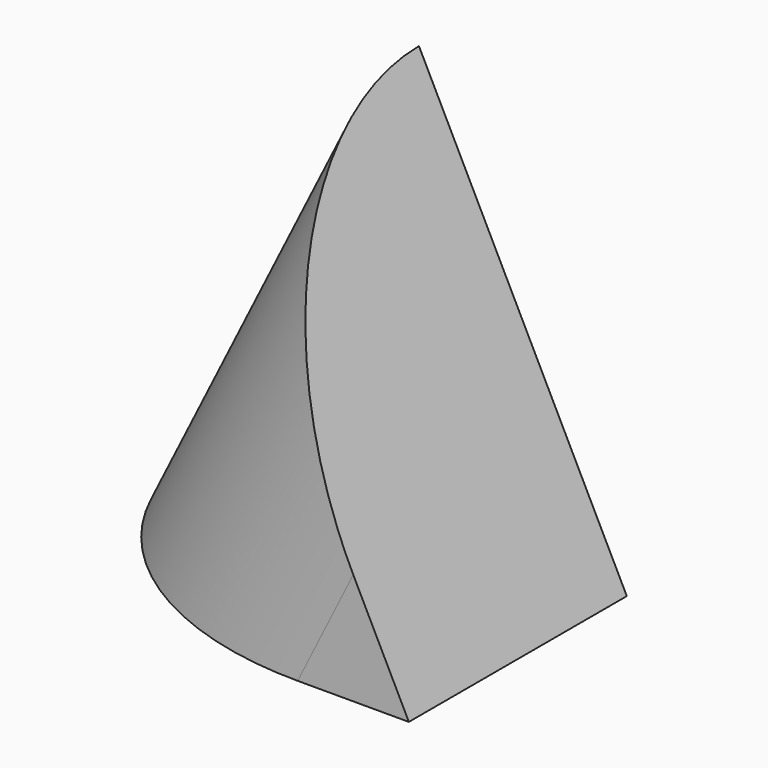
from build123d import *

# Parameters (mm, degrees)
F1_DEPTH = 100
F2_R     = 99.99999


# Not quite as in the source:
# - a fillet or chamfer is up to 0.001 mm smaller than in the source, because OpenCascade refuses the exact size


with BuildPart() as f1:
    # F0 (on Front) → F1 (new body)
    with BuildSketch(Plane.XZ):
        Polygon((76.2885510921, -76.5387266874), (0, 76.4059126377), (-76.2803032994, -76.5387266874), align=None)
    extrude(amount=F1_DEPTH)

    # F2 (radius 100 in the source; OpenCascade refuses exactly that, so slightly less here)
    f2_edges = [f1.edges().sort_by_distance(p)[0] for p in [
        (-38.140152, -100, -0.066407),
    ]]
    fillet(f2_edges, radius=F2_R)


solid = f1.part
